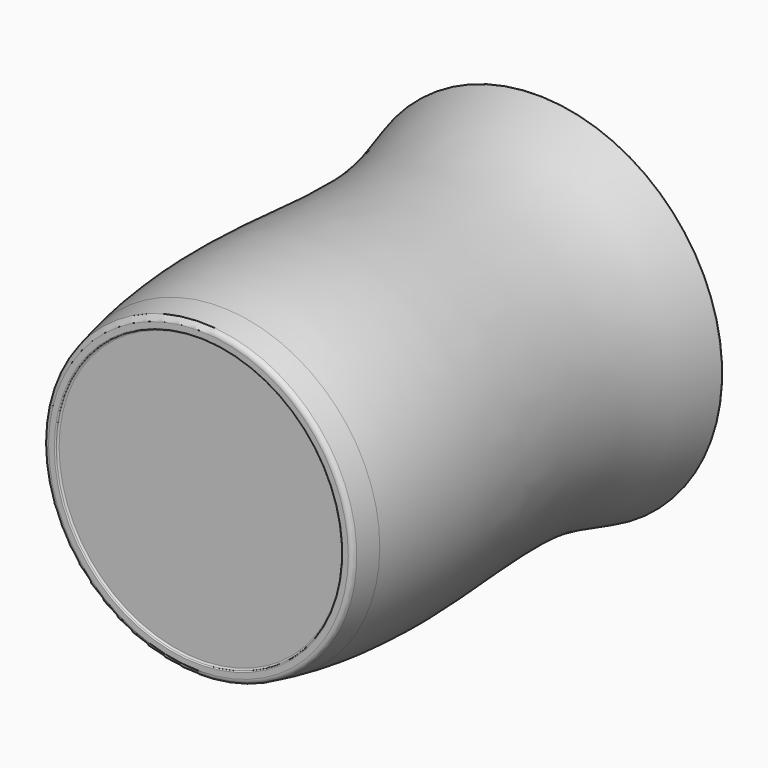
from build123d import *


with BuildPart() as f1:
    # F0 (on Top) → F1 (revolve)
    with BuildSketch(Plane.XY):
        with BuildLine():
            Line((1.3461475165, -25.5006056753), (28.0461475165, -25.5006056753))
            Line((28.0461475165, -25.5006056753), (28.0461475165, -23.0006056753))
            Line((28.0461475165, -23.0006056753), (2.5060778017, -23.0004777587))
            ThreePointArc((2.5060778017, -23.0004777587), (1.2098918631, -22.5235916891), (0.5318353044, -21.3203636915))
            add(Edge.make_bspline(
                [(0.5318353044, -21.3203636915), (-0.8150158739, -13.0079496328), (-2.0915386422, -4.6724136075), (-2.2540024722, 4.0293930826)],
                knots=[0.0306467394, 0.0306467394, 0.0306467394, 0.0306467394, 0.4854691574, 0.4854691574, 0.4854691574, 0.4854691574], degree=3))
            add(Edge.make_bspline(
                [(-2.2540024674, 4.0293931392), (-2.9491607775, -4.0834100782), (-2.6459138796, -14.1064758874), (-2.243888431, -19.5448130064), (-2.1288460014, -20.9459457324)],
                knots=[0.5854099201, 0.5854099201, 0.5854099201, 0.5854099201, 0.8471807154, 0.9488403469, 0.9488403469, 0.9488403469, 0.9488403469], degree=3))
            add(Edge.make_bspline(
                [(-1.2046905869, -25.2221721119), (-1.5202547504, -23.8333295194), (-1.8331186129, -22.4313432856), (-2.1288460014, -20.9459457326)],
                knots=[0.0153515284, 0.0153515284, 0.0153515284, 0.0153515284, 0.0974228675, 0.0974228675, 0.0974228675, 0.0974228675], degree=3))
            ThreePointArc((-1.2046905869, -25.2221721119), (-0.8534177166, -25.7821318862), (-0.2295453084, -26.0006056753))
            Line((-0.2295453084, -26.0006056753), (-0.1538524835, -26.0006056753))
            Line((-0.1538524835, -26.0006056753), (0.0461475165, -26.0006056753))
            Line((0.0461475165, -26.0006056753), (0.8461475165, -26.0006056753))
            ThreePointArc((0.8461475165, -26.0006056753), (0.9875688728, -25.9420270316), (1.0461475165, -25.8006056753))
            ThreePointArc((1.0461475165, -25.8006056753), (1.1340154822, -25.588473641), (1.3461475165, -25.5006056753))
        make_face()
        with BuildLine():
            add(Edge.make_bspline(
                [(-2.2540024674, 4.0293931392), (-2.9491607775, -4.0834100782), (-2.6459138796, -14.1064758874), (-2.243888431, -19.5448130064), (-2.1288460014, -20.9459457324)],
                knots=[0.5854099201, 0.5854099201, 0.5854099201, 0.5854099201, 0.8471807154, 0.9488403469, 0.9488403469, 0.9488403469, 0.9488403469], degree=3))
            add(Edge.make_bspline(
                [(-2.2540024738, 4.0293931678), (-2.4377943101, 13.8735603402), (-1.1958233968, 24.1864774613), (0.0461475165, 34.4993945825)],
                knots=[0.4854691589, 0.4854691589, 0.4854691589, 0.4854691589, 1, 1, 1, 1], degree=3))
            add(Edge.make_bspline(
                [(-5.9007344191, 53.8806275867), (-3.2431522106, 47.9075504763), (-0.5989279583, 41.9249819709), (0.0461475165, 34.4993945825)],
                knots=[0.0017323014, 0.0017323014, 0.0017323014, 0.0017323014, 0.263245612, 0.263245612, 0.263245612, 0.263245612], degree=3))
            ThreePointArc((-5.9007344191, 53.8806275867), (-5.9745150639, 53.9670466848), (-6.0834640006, 53.9993262949))
            Line((-6.0834640006, 53.9993262949), (-6.6823353722, 53.9993262949))
            ThreePointArc((-6.6823353722, 53.9993262949), (-6.8433010525, 53.9180278103), (-6.873404074, 53.7402267925))
            add(Edge.make_bspline(
                [(-2.1288460014, -20.9459457326), (-2.4260388398, -19.4531874284), (-3.5716634781, -12.998246958), (-4.7483602147, 4.4755185853), (-1.2939239656, 34.5036509373), (-5.154538411, 47.8140313282), (-6.873404074, 53.7402267925)],
                knots=[0.0974228675, 0.0974228675, 0.0974228675, 0.0974228675, 0.1799009035, 0.4350204397, 0.748453522, 1, 1, 1, 1], degree=3))
        make_face()
    revolve(axis=Axis((28.0461475165, -25.7506056753, 0), (0, 1, 0)))


solid = f1.part
